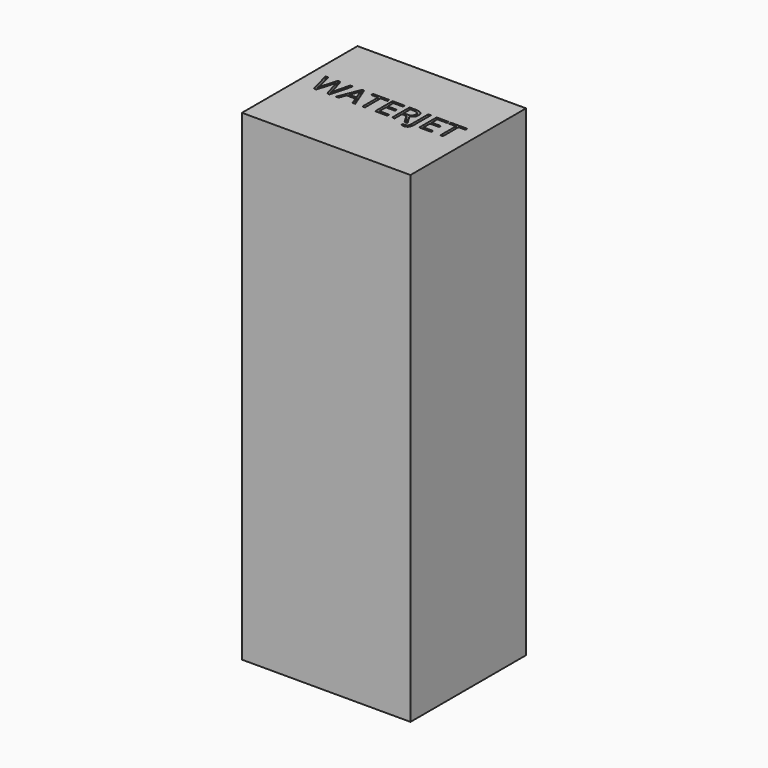
from build123d import *

# Parameters (mm, degrees)
F0_W         = 700
F0_H         = 600
F1_DEPTH     = 2000
F2_TEXT_SIZE = 126.9031857857
F3_DEPTH     = 25


# Not quite as in the source:
# - Text() gives the source's letters only with a copy of the font that has no kerning and outlines rounded to 1/6400 em; it was checked with that copy


with BuildPart() as f1:
    # F0 (on Top) → F1 (new body)
    with BuildSketch(Plane.XY):
        Rectangle(F0_W, F0_H)
    extrude(amount=F1_DEPTH)

    # F2 (on face) → F3 (cut)
    with BuildSketch(Plane.XY.offset(2000)):
        with Locations((-300, -21.5407689836)):
            Text('WATERJET', F2_TEXT_SIZE, font='Open Sans', text_align=(TextAlign.LEFT, TextAlign.BOTTOM))
    extrude(amount=-F3_DEPTH, mode=Mode.SUBTRACT)


solid = f1.part
